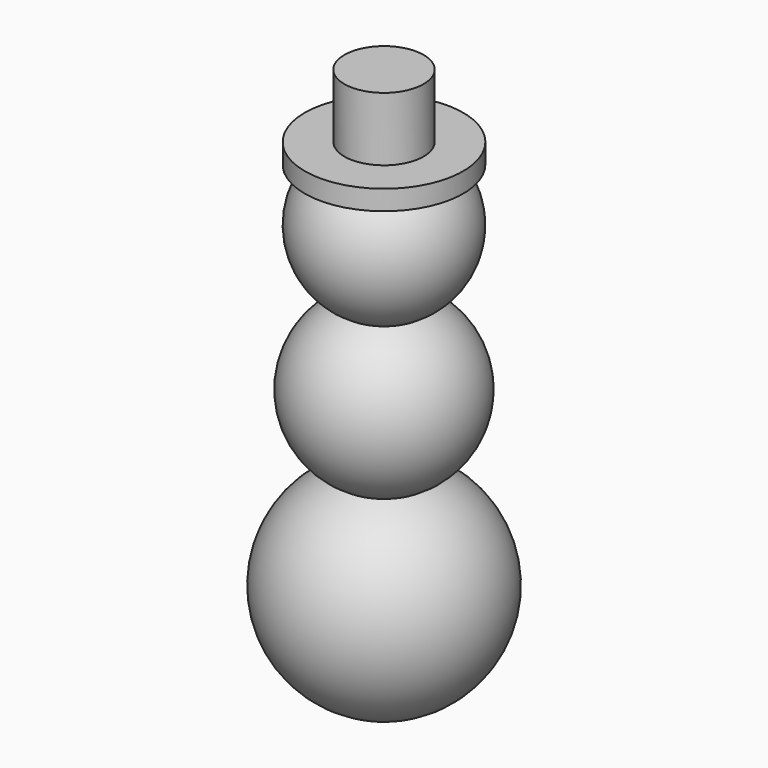
from build123d import *

# Parameters (mm, degrees)
F0_R = 3.9452510547
F1_W = 12.7
F1_H = 20.4561264838


# Not quite as in the source:
# - the program builds the solid bodies; features that only make, move or delete a surface that nothing else refers to are left out


with BuildPart() as f2:
    # F0 (on Front) → F2 (revolve)
    with BuildSketch(Plane.XZ):
        with BuildLine():
            ThreePointArc((0, 71.7677), (-24.5323286084, 52.9498617307), (-12.714626341, 24.3791057518))
            ThreePointArc((-12.714626341, 24.3791057518), (-8.7732416217, 26.0582568814), (-4.6188620822, 27.1047714123))
            ThreePointArc((-4.6188620822, 27.1047714123), (-6.538891729, 30.4166180357), (-6.3411390434, 34.2396712366))
            ThreePointArc((-6.3411390434, 34.2396712366), (-4.6071647855, 29.5343692183), (0, 27.5543271861))
            Line((0, 27.5543271861), (0, 40.2543271861))
            Line((0, 40.2543271861), (-1.7050582101, 40.2543271861))
            Line((-1.7050582101, 40.2543271861), (0, 43.2075746357))
            Line((0, 43.2075746357), (0, 71.7677))
        make_face()
        with Locations((-9.0252510547, 49.9191674486)):
            Circle(F0_R, mode=Mode.SUBTRACT)
    revolve(axis=Axis((0, 0, -8.89), (0, 0, -1)))


with BuildPart() as f2b:
    # F0 (on Front) → F2, piece 2 (revolve)
    with BuildSketch(Plane.XZ):
        with BuildLine():
            Line((0, -20.9677), (0, 20.9677))
            ThreePointArc((0, 20.9677), (-6.5821617307, 21.8353713916), (-12.714626341, 24.3791057518))
            ThreePointArc((-12.714626341, 24.3791057518), (-27.4895738801, 0.5708310965), (-13.7157117337, -23.8302700758))
            ThreePointArc((-13.7157117337, -23.8302700758), (-7.0056237374, -21.6909703998), (0, -20.9677))
        make_face()
    revolve(axis=Axis((0, 0, -8.89), (0, 0, -1)))


with BuildPart() as f2c:
    # F0 (on Front) → F2, piece 3 (revolve)
    with BuildSketch(Plane.XZ):
        with BuildLine():
            Line((0, -89.5477), (0, -27.4955))
            ThreePointArc((0, -27.4955), (-7.0984973544, -26.5633931485), (-13.7157117337, -23.8302700758))
            ThreePointArc((-13.7157117337, -23.8302700758), (-33.5667296002, -62.2633237374), (0, -89.5477))
        make_face()
    revolve(axis=Axis((0, 0, -8.89), (0, 0, -1)))


with BuildPart() as f3:
    # F1 (on Front) → F3 (revolve)
    with BuildSketch(Plane.XZ):
        with Locations((-6.35, 80.0780632419)):
            Rectangle(F1_W, F1_H)
        Polygon((0, 63.5), (0, 69.85), (-12.7, 69.85), (-25.4, 69.85), (-25.4, 63.5), align=None)
    revolve(axis=Axis((0, 0, 66.675), (0, 0, -1)))


solid = Compound([f2.part, f2b.part, f2c.part, f3.part])
